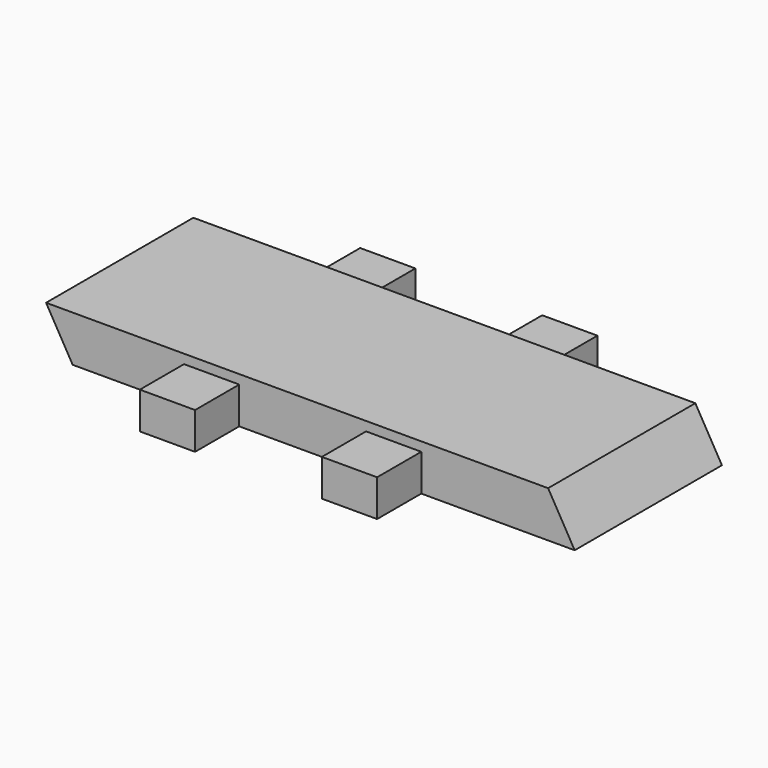
from build123d import *

# Parameters (mm, degrees)
F1_DEPTH    = 6.35
F0_W        = 7.62
F0_H        = 7.62
F2_DEPTH    = 5.08
F3_T1_DEPTH = 63.3815233811


# Not quite as in the source:
# - a fillet or chamfer that OpenCascade refuses, or shapes differently, is made with other operations: its cross-section is extruded or revolved along the edge and cut away or added


with BuildPart() as f1:
    # F0 (on Top) → F1 (new body)
    with BuildSketch(Plane.XY):
        Polygon((-23.7489993078, -7.62), (-41.2495993078, -7.62), (-41.2495993078, -33.02), (-21.6407993078, -33.02), (-14.0207993078, -33.02), (3.4798006922, -33.02), (11.0998006922, -33.02), (32.8422006922, -33.02), (32.8422006922, -7.62), (8.9916006922, -7.62), (1.3716006922, -7.62), (-16.1289993078, -7.62), align=None)
    extrude(amount=F1_DEPTH)

    # F0 (on Top) → F2 (join)
    with BuildSketch(Plane.XY):
        with Locations((-19.9389993078, -3.81)):
            Rectangle(F0_W, F0_H)
        with Locations((-17.8307993078, -36.83)):
            Rectangle(F0_W, F0_H)
        with Locations((7.2898006922, -36.83)):
            Rectangle(F0_W, F0_H)
        with Locations((5.1816006922, -3.81)):
            Rectangle(F0_W, F0_H)
    extrude(amount=F2_DEPTH)

    # F3: chamfer of 7.3406 x 4.238097386 on 2 edges, made by hand

    # F3_s2 → F3_t1 (cut)
    with BuildSketch(Plane.XZ.offset(-11.3707616906)):
        Polygon((28.6041033062, 6.35), (32.8422006922, -0.9906), (32.8422006922, 6.35), align=None)
        Polygon((-41.2495993078, 7.3406), (-37.0115019218, 0), (-41.2495993078, 0), align=None)
    extrude(amount=F3_T1_DEPTH, mode=Mode.SUBTRACT)


solid = f1.part
